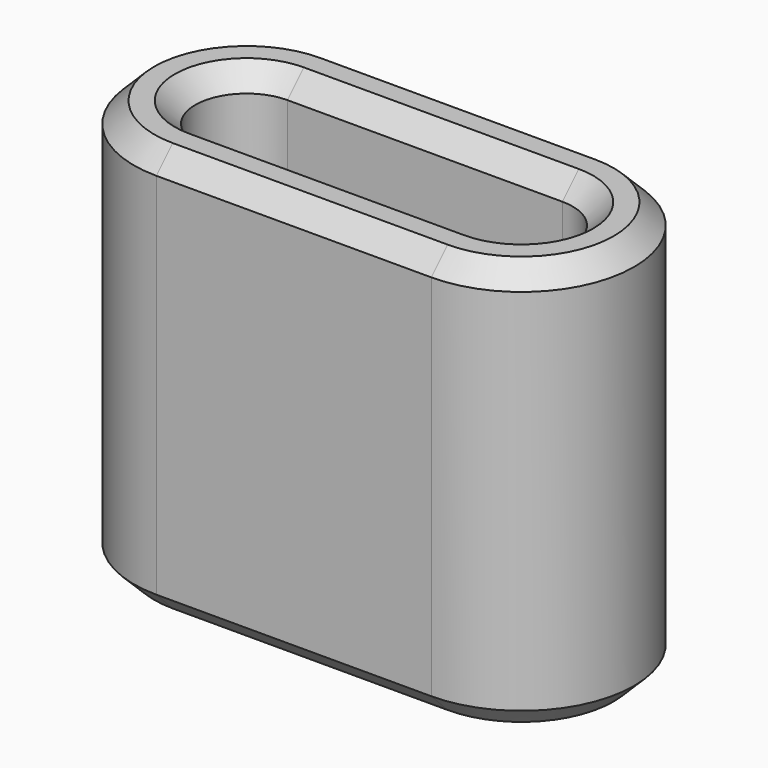
from build123d import *

# Parameters (mm, degrees)
F1_DEPTH = 10
F2_SIZE  = 0.5


# Not quite as in the source:
# - ends of sketch curves that miss each other by under 0.0002 mm in the source are joined


with BuildPart() as f1:
    # F0 (on Top) → F1 (new body)
    with BuildSketch(Plane.XY):
        with BuildLine():
            Line((3.3542521534, 2.75), (-3.3557469528, 2.75))
            ThreePointArc((-3.3557469528, 2.75), (-6.1057473997, -4.469e-07), (-3.3557469528, -2.7500008938))
            Line((-3.3557469528, -2.7500008938), (3.3542521534, -2.75))
            ThreePointArc((3.3542521534, -2.75), (6.1042526003, -4.469e-07), (3.3542521534, 2.75))
        make_face()
        with BuildLine():
            Line((-3.3557469528, 1.25), (3.3542521534, 1.25))
            ThreePointArc((3.3542521534, 1.25), (4.6042523768, 0.000746953), (3.3557469528, -1.25))
            Line((3.3557469528, -1.25), (-3.3542521534, -1.25))
            ThreePointArc((-3.3542521534, -1.25), (-4.6057471763, -0.0007478467), (-3.3557469528, 1.25))
        make_face(mode=Mode.SUBTRACT)
    extrude(amount=F1_DEPTH)

    # F2
    f2_edges = [f1.edges().sort_by_distance(p)[0] for p in [
        (-0.000747, -2.75, 10),
        (6.104253, 0, 10),
        (-0.000747, 2.75, 10),
        (-6.105747, 0, 10),
        (-0.000747, 1.25, 10),
        (4.604252, 0.000747, 10),
        (0.000747, -1.25, 10),
        (-4.605747, -0.000748, 10),
        (-0.000747, -2.75, 0),
        (6.104253, 0, 0),
        (-0.000747, 2.75, 0),
        (-6.105747, 0, 0),
        (-0.000747, 1.25, 0),
        (4.604252, 0.000747, 0),
        (0.000747, -1.25, 0),
        (-4.605747, -0.000748, 0),
    ]]
    chamfer(f2_edges, length=F2_SIZE)


solid = f1.part
